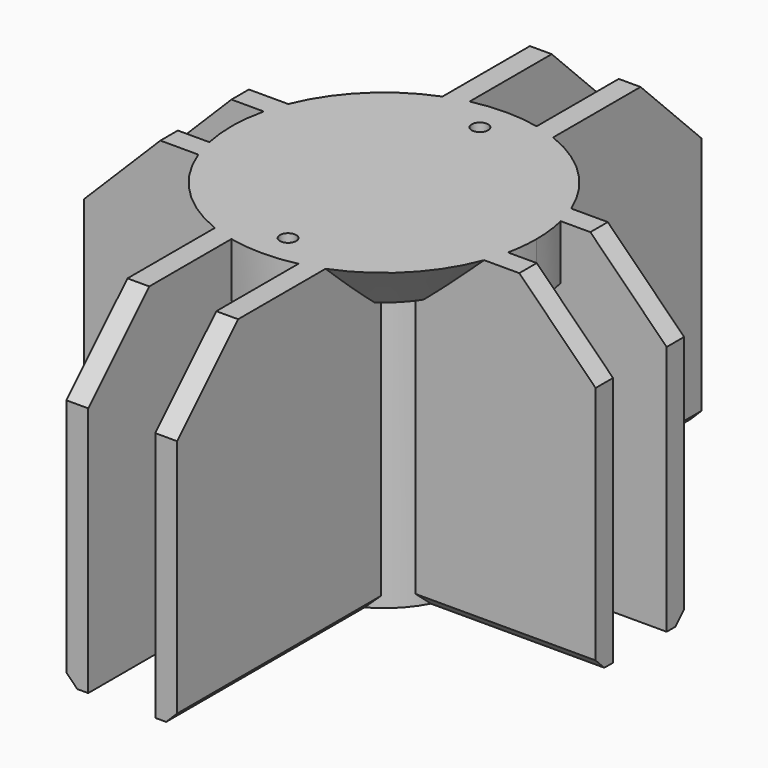
from build123d import *

# Parameters (mm, degrees)
F1_DEPTH = 25
F2_W     = 6.15
F2_H     = 2
F2_W_2   = 2
F2_H_2   = 6.15
F3_DEPTH = 25
F5_DEPTH = 5
F6_R     = 0.75
F7_DEPTH = 5
F8_DEPTH = 5
F9_SIZE  = 7
F10_SIZE = 4.99999
F11_SIZE = 1


# Not quite as in the source:
# - a fillet or chamfer is up to 0.001 mm smaller than in the source, because OpenCascade refuses the exact size


with BuildPart() as f1:
    # F0 (on Top) → F1 (new body)
    with BuildSketch(Plane.XY):
        with BuildLine():
            Line((5.5211611295, 29.3387952344), (-4.6288388705, 29.3387952344))
            Line((-4.6288388705, 29.3387952344), (-4.6288388705, 5.9433882713))
            ThreePointArc((-4.6288388705, 5.9433882713), (-5.4099272548, 5.2703597245), (-6.1025520558, 4.5065944634))
            Line((-6.1025520558, 4.5065944634), (-23.141437278, 4.5065944634))
            Line((-23.141437278, 4.5065944634), (-23.141437278, -5.6434055366))
            Line((-23.141437278, -5.6434055366), (-6.3576590277, -5.6434055366))
            ThreePointArc((-6.3576590277, -5.6434055366), (-5.5589979581, -6.5937343191), (-4.6288388705, -7.4157978024))
            Line((-4.6288388705, -7.4157978024), (-4.6288388705, -30.8112047656))
            Line((-4.6288388705, -30.8112047656), (5.5211611295, -30.8112047656))
            Line((5.5211611295, -30.8112047656), (5.5211611295, -7.4157978024))
            ThreePointArc((5.5211611295, -7.4157978024), (6.4513202171, -6.5937343191), (7.2499812866, -5.6434055366))
            Line((7.2499812866, -5.6434055366), (23.7822366705, -5.6434055366))
            Line((23.7822366705, -5.6434055366), (23.7822366705, 4.5065944634))
            Line((23.7822366705, 4.5065944634), (6.9948743147, 4.5065944634))
            ThreePointArc((6.9948743147, 4.5065944634), (6.3022495138, 5.2703597245), (5.5211611295, 5.9433882713))
            Line((5.5211611295, 5.9433882713), (5.5211611295, 29.3387952344))
        make_face()
        with BuildLine():
            Line((-2.6288388705, 4.8639394003), (-2.6288388705, 27.3387952344))
            Line((-2.6288388705, 27.3387952344), (3.5211611295, 27.3387952344))
            Line((3.5211611295, 27.3387952344), (3.5211611295, 4.8639394003))
            ThreePointArc((3.5211611295, 4.8639394003), (4.8949803528, 3.8491247969), (5.9508403063, 2.5065944634))
            Line((5.9508403063, 2.5065944634), (21.7822366705, 2.5065944634))
            Line((21.7822366705, 2.5065944634), (21.7822366705, -3.6434055366))
            Line((21.7822366705, -3.6434055366), (6.1352228584, -3.6434055366))
            ThreePointArc((6.1352228584, -3.6434055366), (5.0303928567, -5.1861552316), (3.5211611295, -6.3363489315))
            Line((3.5211611295, -6.3363489315), (3.5211611295, -28.8112047656))
            Line((3.5211611295, -28.8112047656), (-2.6288388705, -28.8112047656))
            Line((-2.6288388705, -28.8112047656), (-2.6288388705, -6.3363489315))
            ThreePointArc((-2.6288388705, -6.3363489315), (-4.1380705978, -5.1861552316), (-5.2429005995, -3.6434055366))
            Line((-5.2429005995, -3.6434055366), (-21.141437278, -3.6434055366))
            Line((-21.141437278, -3.6434055366), (-21.141437278, 2.5065944634))
            Line((-21.141437278, 2.5065944634), (-5.0585180473, 2.5065944634))
            ThreePointArc((-5.0585180473, 2.5065944634), (-4.0026580939, 3.8491247969), (-2.6288388705, 4.8639394003))
        make_face(mode=Mode.SUBTRACT)
    extrude(amount=-F1_DEPTH)

    # F2 (on face) → F3 (cut, through all)
    with BuildSketch(Plane.XY):
        with Locations((0.4461611295, 28.3387952344)):
            Rectangle(F2_W, F2_H)
        with Locations((-22.141437278, -0.5684055366)):
            Rectangle(F2_W_2, F2_H_2)
        with Locations((22.7822366705, -0.5684055366)):
            Rectangle(F2_W_2, F2_H_2)
        with Locations((0.4461611295, -29.8112047656)):
            Rectangle(F2_W, F2_H)
    extrude(amount=-F3_DEPTH, mode=Mode.SUBTRACT)

    # F4 (on Top) → F5 (join)
    with BuildSketch(Plane.XY):
        with BuildLine():
            Line((3.5211611295, 4.8639394003), (3.5211611295, 12.9219201057))
            ThreePointArc((3.5211611295, 12.9219201057), (0.4461611295, 13.2637952344), (-2.6288388705, 12.9219201057))
            Line((-2.6288388705, 12.9219201057), (-2.6288388705, 4.8639394003))
            ThreePointArc((-2.6288388705, 4.8639394003), (-4.0026580939, 3.8491247969), (-5.0585180473, 2.5065944634))
            Line((-5.0585180473, 2.5065944634), (-13.1730992455, 2.5065944634))
            ThreePointArc((-13.1730992455, 2.5065944634), (-13.5527822586, -0.5642047132), (-13.2486621142, -3.6434055366))
            Line((-13.2486621142, -3.6434055366), (-5.2429005995, -3.6434055366))
            ThreePointArc((-5.2429005995, -3.6434055366), (-4.1380705978, -5.1861552316), (-2.6288388705, -6.3363489315))
            Line((-2.6288388705, -6.3363489315), (-2.6288388705, -14.3943296369))
            ThreePointArc((-2.6288388705, -14.3943296369), (0.4461611295, -14.7362047656), (3.5211611295, -14.3943296369))
            Line((3.5211611295, -14.3943296369), (3.5211611295, -6.3363489315))
            ThreePointArc((3.5211611295, -6.3363489315), (5.0303928567, -5.1861552316), (6.1352228584, -3.6434055366))
            Line((6.1352228584, -3.6434055366), (14.1409843732, -3.6434055366))
            ThreePointArc((14.1409843732, -3.6434055366), (14.3696579139, -2.1977920171), (14.4461611295, -0.7362047656))
            ThreePointArc((14.4461611295, -0.7362047656), (14.350650427, 0.8963323321), (14.0654215044, 2.5065944634))
            Line((14.0654215044, 2.5065944634), (5.9508403063, 2.5065944634))
            ThreePointArc((5.9508403063, 2.5065944634), (4.8949803528, 3.8491247969), (3.5211611295, 4.8639394003))
        make_face()
        with BuildLine():
            ThreePointArc((13.5579642318, -5.6434055366), (13.8867267431, -4.6542649982), (14.1409843732, -3.6434055366))
            Line((14.1409843732, -3.6434055366), (6.1352228584, -3.6434055366))
            ThreePointArc((6.1352228584, -3.6434055366), (5.0303928567, -5.1861552316), (3.5211611295, -6.3363489315))
            Line((3.5211611295, -6.3363489315), (3.5211611295, -14.3943296369))
            ThreePointArc((3.5211611295, -14.3943296369), (4.5325724418, -14.1265461573), (5.5211611295, -13.783977564))
            Line((5.5211611295, -13.783977564), (5.5211611295, -7.4157978024))
            ThreePointArc((5.5211611295, -7.4157978024), (6.4513202171, -6.5937343191), (7.2499812866, -5.6434055366))
            Line((7.2499812866, -5.6434055366), (13.5579642318, -5.6434055366))
        make_face()
        with BuildLine():
            Line((-4.6288388705, 5.9433882713), (-4.6288388705, 12.3115680329))
            ThreePointArc((-4.6288388705, 12.3115680329), (-9.3893111671, 9.2269014119), (-12.5350967543, 4.5065944634))
            Line((-12.5350967543, 4.5065944634), (-6.1025520558, 4.5065944634))
            ThreePointArc((-6.1025520558, 4.5065944634), (-5.4099272548, 5.2703597245), (-4.6288388705, 5.9433882713))
        make_face()
        with BuildLine():
            Line((-2.6288388705, 4.8639394003), (-2.6288388705, 12.9219201057))
            ThreePointArc((-2.6288388705, 12.9219201057), (-3.6402501828, 12.6541366261), (-4.6288388705, 12.3115680329))
            Line((-4.6288388705, 12.3115680329), (-4.6288388705, 5.9433882713))
            ThreePointArc((-4.6288388705, 5.9433882713), (-5.4099272548, 5.2703597245), (-6.1025520558, 4.5065944634))
            Line((-6.1025520558, 4.5065944634), (-12.5350967543, 4.5065944634))
            ThreePointArc((-12.5350967543, 4.5065944634), (-12.8916382733, 3.5185698574), (-13.1730992455, 2.5065944634))
            Line((-13.1730992455, 2.5065944634), (-5.0585180473, 2.5065944634))
            ThreePointArc((-5.0585180473, 2.5065944634), (-4.0026580939, 3.8491247969), (-2.6288388705, 4.8639394003))
        make_face()
        with BuildLine():
            ThreePointArc((13.4274190132, 4.5065944634), (10.281633426, 9.2269014119), (5.5211611295, 12.3115680329))
            Line((5.5211611295, 12.3115680329), (5.5211611295, 5.9433882713))
            ThreePointArc((5.5211611295, 5.9433882713), (6.3022495138, 5.2703597245), (6.9948743147, 4.5065944634))
            Line((6.9948743147, 4.5065944634), (13.4274190132, 4.5065944634))
        make_face()
        with BuildLine():
            Line((5.5211611295, 5.9433882713), (5.5211611295, 12.3115680329))
            ThreePointArc((5.5211611295, 12.3115680329), (4.5325724418, 12.6541366261), (3.5211611295, 12.9219201057))
            Line((3.5211611295, 12.9219201057), (3.5211611295, 4.8639394003))
            ThreePointArc((3.5211611295, 4.8639394003), (4.8949803528, 3.8491247969), (5.9508403063, 2.5065944634))
            Line((5.9508403063, 2.5065944634), (14.0654215044, 2.5065944634))
            ThreePointArc((14.0654215044, 2.5065944634), (13.7839605322, 3.5185698574), (13.4274190132, 4.5065944634))
            Line((13.4274190132, 4.5065944634), (6.9948743147, 4.5065944634))
            ThreePointArc((6.9948743147, 4.5065944634), (6.3022495138, 5.2703597245), (5.5211611295, 5.9433882713))
        make_face()
        with BuildLine():
            ThreePointArc((5.5211611295, -13.783977564), (10.4089508996, -10.5719975652), (13.5579642318, -5.6434055366))
            Line((13.5579642318, -5.6434055366), (7.2499812866, -5.6434055366))
            ThreePointArc((7.2499812866, -5.6434055366), (6.4513202171, -6.5937343191), (5.5211611295, -7.4157978024))
            Line((5.5211611295, -7.4157978024), (5.5211611295, -13.783977564))
        make_face()
        with BuildLine():
            Line((-6.3576590277, -5.6434055366), (-12.6656419728, -5.6434055366))
            ThreePointArc((-12.6656419728, -5.6434055366), (-9.5166286406, -10.5719975652), (-4.6288388705, -13.783977564))
            Line((-4.6288388705, -13.783977564), (-4.6288388705, -7.4157978024))
            ThreePointArc((-4.6288388705, -7.4157978024), (-5.5589979581, -6.5937343191), (-6.3576590277, -5.6434055366))
        make_face()
        with BuildLine():
            Line((-5.2429005995, -3.6434055366), (-13.2486621142, -3.6434055366))
            ThreePointArc((-13.2486621142, -3.6434055366), (-12.9944044841, -4.6542649982), (-12.6656419728, -5.6434055366))
            Line((-12.6656419728, -5.6434055366), (-6.3576590277, -5.6434055366))
            ThreePointArc((-6.3576590277, -5.6434055366), (-5.5589979581, -6.5937343191), (-4.6288388705, -7.4157978024))
            Line((-4.6288388705, -7.4157978024), (-4.6288388705, -13.783977564))
            ThreePointArc((-4.6288388705, -13.783977564), (-3.6402501828, -14.1265461573), (-2.6288388705, -14.3943296369))
            Line((-2.6288388705, -14.3943296369), (-2.6288388705, -6.3363489315))
            ThreePointArc((-2.6288388705, -6.3363489315), (-4.1380705978, -5.1861552316), (-5.2429005995, -3.6434055366))
        make_face()
    extrude(amount=F5_DEPTH)

    # F6 (on face) → F7 (cut, through all)
    with BuildSketch(Plane.XY.offset(5)):
        with Locations((0.4461611295, 10.2637952344)):
            Circle(F6_R)
        with Locations((0.4461611295, -11.7362047656)):
            Circle(F6_R)
    extrude(amount=-F7_DEPTH, mode=Mode.SUBTRACT)

    # F8 (add): faces of the model
    f8_faces = [f1.faces().sort_by_distance(p)[0] for p in [
        (-3.6349246548, 20.9904665399, 0),
        (4.5272469138, 20.9904665399, 0),
        (18.7764211463, 3.5172058862, 0),
        (18.8278982695, -4.6532031137, 0),
        (-18.0099019482, 3.5169457421, 0),
        (-18.0613729447, -4.6529604993, 0),
        (-3.6349246548, -22.4628760711, 0),
        (4.5272469138, -22.4628760711, 0),
    ]]
    extrude(f8_faces, amount=F8_DEPTH)

    # F9
    f9_edges = [f1.edges().sort_by_distance(p)[0] for p in [
        (-23.141437, 3.506594, 5),
        (-23.141437, -4.643406, 5),
        (-3.628839, -30.811205, 5),
        (4.521161, -30.811205, 5),
        (23.782237, -4.643406, 5),
        (23.782237, 3.506594, 5),
        (-3.628839, 29.338795, 5),
        (4.521161, 29.338795, 5),
    ]]
    chamfer(f9_edges, length=F9_SIZE)

    # F10 (size 5 in the source; OpenCascade refuses exactly that, so slightly less here)
    f10_edges = [f1.edges().sort_by_distance(p)[0] for p in [
        (10.281633, 9.226901, 0),
        (-9.389311, 9.226901, 0),
        (10.408951, -10.571998, 0),
        (-9.516629, -10.571998, 0),
    ]]
    chamfer(f10_edges, length=F10_SIZE)

    # F11
    f11_edges = [f1.edges().sort_by_distance(p)[0] for p in [
        (15.388555, 4.506594, -25),
        (5.521161, 17.641092, -25),
        (-4.628839, 17.641092, -25),
        (-14.621995, 4.506594, -25),
        (-14.749548, -5.643406, -25),
        (-4.628839, -19.113501, -25),
        (5.521161, -19.113501, -25),
        (15.516109, -5.643406, -25),
    ]]
    chamfer(f11_edges, length=F11_SIZE)


solid = f1.part
